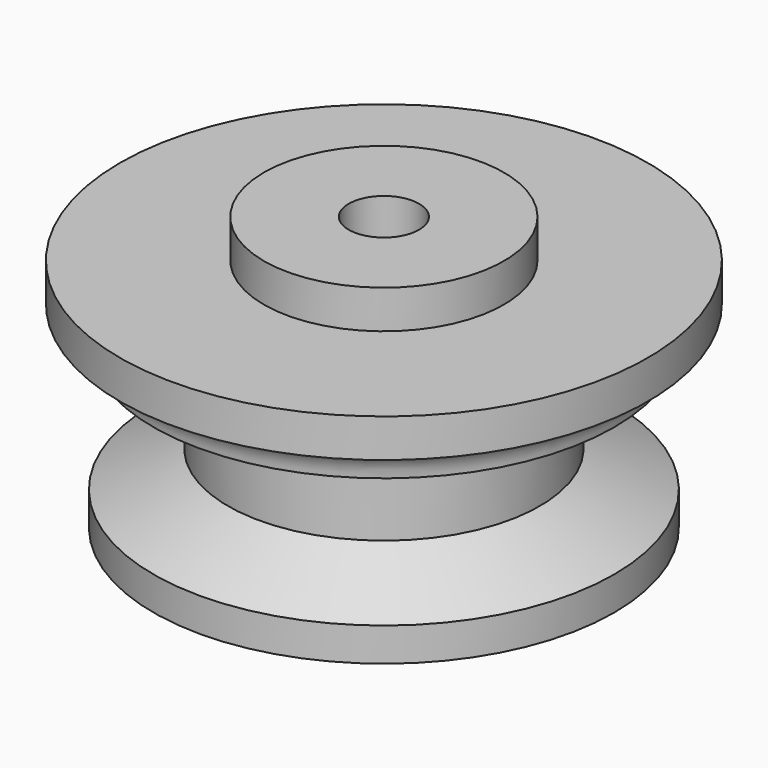
from build123d import *

# Parameters (mm, degrees)
F3_R     = 1.04999
F4_R     = 1.1
F5_DEPTH = 8.551


# Not quite as in the source:
# - a fillet or chamfer is up to 0.001 mm smaller than in the source, because OpenCascade refuses the exact size


with BuildPart() as f2:
    # F1 (on Front) → F2 (revolve)
    with BuildSketch(Plane.XZ):
        Polygon((-7.2, 0), (0, 0), (0, 8.55), (-3.75, 8.55), (-3.75, 7.35), (-8.25, 7.35), (-8.25, 6.15), (-7.2, 6.15), (-7.2, 5.1), (-4.875, 3.975), (-4.875, 2.175), (-7.2, 1.05), align=None)
    revolve(axis=Axis((0, 0, 4.275), (0, 0, -1)))

    # F3 (radius 1.05 in the source; OpenCascade refuses exactly that, so slightly less here)
    f3_edges = [f2.edges().sort_by_distance(p)[0] for p in [
        (7.2, 0, 6.15),
    ]]
    fillet(f3_edges, radius=F3_R)

    # F4 (on face) → F5 (cut, through all)
    with BuildSketch(Plane.XY.offset(8.55)):
        Circle(F4_R)
    extrude(amount=-F5_DEPTH, mode=Mode.SUBTRACT)


solid = f2.part
